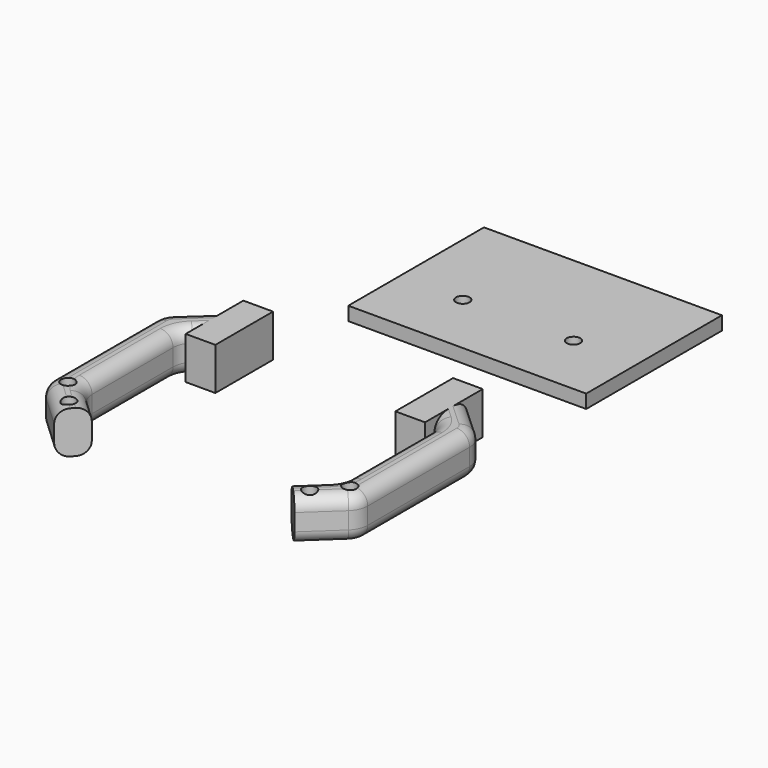
from build123d import *

# Parameters (mm, degrees)
F0_W           = 56.1
F0_H           = 40
F0_R           = 1.6
F1_DEPTH       = 3.2
F2_R           = 1.6
F3_DEPTH       = 10
F4_T1_DEPTH    = 23.8781775711
F4_T3_DEPTH    = 30
F4_T5_DEPTH    = 17.5
F4_T7_DEPTH    = 14.4606096023
F4_T10_ANGLE   = 47.5323400186
F4_T12_ANGLE   = 47.5323400186
F4_T14_ANGLE   = 46.9408390922
F4_T16_ANGLE   = 46.9408390922
F4_T18_ANGLE   = 47.5323400186
F4_T20_ANGLE   = 47.5323400186
F4_T24_DEPTH   = 8.0105146464
F4_T29_DEPTH   = 8.0105146464
F4_T34_DEPTH   = 17.5
F4_T39_DEPTH   = 17.5
F4_T42_ANGLE   = 46.9408390922
F4_T44_ANGLE   = 46.9408390922
F4_2_T1_DEPTH  = 23.8781775711
F4_2_T3_DEPTH  = 30
F4_2_T5_DEPTH  = 14.4606096023
F4_2_T7_DEPTH  = 17.5
F4_2_T12_DEPTH = 8.0105146464
F4_2_T17_DEPTH = 8.0105146464
F4_2_T20_ANGLE = 47.5323400186
F4_2_T22_ANGLE = 47.5323400186
F4_2_T24_ANGLE = 46.9408390922
F4_2_T26_ANGLE = 46.9408390922
F4_2_T28_ANGLE = 47.5323400186
F4_2_T30_ANGLE = 47.5323400186
F4_2_T34_DEPTH = 17.5
F4_2_T39_DEPTH = 17.5
F4_2_T42_ANGLE = 46.9408390922
F4_2_T44_ANGLE = 46.9408390922


# Not quite as in the source:
# - a fillet or chamfer that OpenCascade refuses, or shapes differently, is made with other operations: its cross-section is extruded or revolved along the edge and cut away or added


with BuildPart() as f1:
    # F0 (on Top) → F1 (new body)
    with BuildSketch(Plane.XY):
        with Locations((-11.1600676847, 12.4215162359)):
            Rectangle(F0_W, F0_H)
        with Locations((-24.2100676847, 7.4215162359)):
            Circle(F0_R, mode=Mode.SUBTRACT)
        with Locations((1.8899323153, 7.4215162359)):
            Circle(F0_R, mode=Mode.SUBTRACT)
    extrude(amount=F1_DEPTH)


with BuildPart() as f3:
    # F2 (on Top) → F3 (new body)
    with BuildSketch(Plane.XY):
        with BuildLine():
            Line((-56.4012295696, -43.395672177), (-56.4012295696, -73.395672177))
            ThreePointArc((-56.4012295696, -73.395672177), (-55.9875586538, -75.387049974), (-54.8149953573, -77.0489177403))
            Line((-54.8149953573, -77.0489177403), (-47.5085042306, -83.8764493159))
            Line((-47.5085042306, -83.8764493159), (-42.7292321277, -78.7619055271))
            Line((-42.7292321277, -78.7619055271), (-47.8149953573, -74.0095273427))
            ThreePointArc((-47.8149953573, -74.0095273427), (-48.9875586538, -72.3476595763), (-49.4012295696, -70.3562817793))
            Line((-49.4012295696, -70.3562817793), (-49.4012295696, -46.4781042082))
            ThreePointArc((-49.4012295696, -46.4781042082), (-48.9772184672, -44.4630792435), (-47.7770993263, -42.7898114614))
            Line((-47.7770993263, -42.7898114614), (-47.4005138328, -42.4451252704))
            Line((-47.4005138328, -42.4451252704), (-47.4005138328, -32.9556399168))
            Line((-47.4005138328, -32.9556399168), (-54.7770993263, -39.7073794302))
            ThreePointArc((-54.7770993263, -39.7073794302), (-55.9772184672, -41.3806472123), (-56.4012295696, -43.395672177))
        make_face()
        with Locations((-47.5562252104, -79.4592574239)):
            Circle(F2_R, mode=Mode.SUBTRACT)
        with Locations((-52.413392812, -73.7146958709)):
            Circle(F2_R, mode=Mode.SUBTRACT)
        Polygon((-47.4005138328, -28.2597062046), (-47.4005138328, -32.9556399168), (-47.4005138328, -42.4451252704), (-47.4005138328, -45.2568237537), (-40.4005138328, -45.2568237537), (-40.4005138328, -28.2597062046), align=None)
    extrude(amount=F3_DEPTH)

    # F4: fillet of radius 3 on 18 edges, made by hand

    # F4_s2 → F4_t1 (cut)
    with BuildSketch(Plane.XZ.offset(46.4781042082)):
        with BuildLine():
            ThreePointArc((-49.4012295696, 7), (-50.279909226, 9.1213203436), (-52.4012295696, 10))
            Line((-52.4012295696, 10), (-49.4012295696, 10))
            Line((-49.4012295696, 10), (-49.4012295696, 7))
        make_face()
        with BuildLine():
            ThreePointArc((-49.4012295696, 3), (-50.279909226, 0.8786796564), (-52.4012295696, 0))
            Line((-52.4012295696, 0), (-49.4012295696, 0))
            Line((-49.4012295696, 0), (-49.4012295696, 3))
        make_face()
    extrude(amount=F4_T1_DEPTH, mode=Mode.SUBTRACT)

    # F4_s4 → F4_t3 (cut)
    with BuildSketch(Plane.XZ.offset(43.395672177)):
        with BuildLine():
            ThreePointArc((-56.4012295696, 7), (-55.5225499131, 9.1213203436), (-53.4012295696, 10))
            Line((-53.4012295696, 10), (-56.4012295696, 10))
            Line((-56.4012295696, 10), (-56.4012295696, 7))
        make_face()
        with BuildLine():
            ThreePointArc((-56.4012295696, 3), (-55.5225499131, 0.8786796564), (-53.4012295696, 0))
            Line((-53.4012295696, 0), (-56.4012295696, 0))
            Line((-56.4012295696, 0), (-56.4012295696, 3))
        make_face()
    extrude(amount=F4_T3_DEPTH, mode=Mode.SUBTRACT)

    # F4_s6 → F4_t5 (cut)
    with BuildSketch(Plane(origin=(9.1732003541, -8.571873144, 0), x_dir=(0, 0, 1), z_dir=(0.7306491127, -0.6827531576, 0))):
        with BuildLine():
            ThreePointArc((3, 93.7208345409), (0.8786796564, 92.8421548845), (0, 90.7208345409))
            Line((0, 90.7208345409), (0, 93.7208345409))
            Line((0, 93.7208345409), (3, 93.7208345409))
        make_face()
        with BuildLine():
            ThreePointArc((7, 93.7208345409), (9.1213203436, 92.8421548845), (10, 90.7208345409))
            Line((10, 90.7208345409), (10, 93.7208345409))
            Line((10, 93.7208345409), (7, 93.7208345409))
        make_face()
    extrude(amount=F4_T5_DEPTH, mode=Mode.SUBTRACT)

    # F4_s8 → F4_t7 (cut)
    with BuildSketch(Plane(origin=(21.9595598259, -20.5200534012, 0), x_dir=(0, 0, 1), z_dir=(-0.7306491127, 0.6827531576, 0))):
        with BuildLine():
            ThreePointArc((3, -86.7208345409), (0.8786796564, -87.5995141973), (0, -89.7208345409))
            Line((0, -89.7208345409), (0, -86.7208345409))
            Line((0, -86.7208345409), (3, -86.7208345409))
        make_face()
        with BuildLine():
            ThreePointArc((7, -86.7208345409), (9.1213203436, -87.5995141973), (10, -89.7208345409))
            Line((10, -89.7208345409), (10, -86.7208345409))
            Line((10, -86.7208345409), (7, -86.7208345409))
        make_face()
    extrude(amount=F4_T7_DEPTH, mode=Mode.SUBTRACT)

    # F4_s9 → F4_t10 (revolve, cut)
    with BuildSketch(Plane(origin=(-49.582592704, -45.3826164738, 0), x_dir=(0, 0, 1), z_dir=(0.7376585493, 0.6751739513, 0))):
        with BuildLine():
            ThreePointArc((3, -7.6935826862), (0.8786796564, -6.8149030298), (0, -4.6935826862))
            Line((0, -4.6935826862), (0, -7.6935826862))
            Line((0, -7.6935826862), (3, -7.6935826862))
        make_face()
    revolve(axis=Axis((-51.4012295696, -43.395672177, 0), (0, 0, 1)), revolution_arc=F4_T10_ANGLE, mode=Mode.SUBTRACT)

    # F4_s11 → F4_t12 (revolve, cut)
    with BuildSketch(Plane(origin=(-49.582592704, -45.3826164738, 0), x_dir=(0, 0, 1), z_dir=(0.7376585493, 0.6751739513, 0))):
        with BuildLine():
            ThreePointArc((7, -7.6935826862), (9.1213203436, -6.8149030298), (10, -4.6935826862))
            Line((10, -4.6935826862), (10, -7.6935826862))
            Line((10, -7.6935826862), (7, -7.6935826862))
        make_face()
    revolve(axis=Axis((-51.4012295696, -43.395672177, 10), (0, 0, 1)), revolution_arc=F4_T12_ANGLE, mode=Mode.SUBTRACT)

    # F4_s13 → F4_t14 (revolve, cut)
    with BuildSketch(Plane(origin=(11.3939282512, -10.6470265351, 0), x_dir=(0, 0, 1), z_dir=(0.7306491127, -0.6827531576, 0))):
        with BuildLine():
            ThreePointArc((3, 86.7208345409), (0.8786796564, 87.5995141973), (0, 89.7208345409))
            Line((0, 89.7208345409), (0, 86.7208345409))
            Line((0, 86.7208345409), (3, 86.7208345409))
        make_face()
    revolve(axis=Axis((-44.4012295696, -70.3562817793, 0), (0, 0, -1)), revolution_arc=F4_T14_ANGLE, mode=Mode.SUBTRACT)

    # F4_s15 → F4_t16 (revolve, cut)
    with BuildSketch(Plane(origin=(11.3939282512, -10.6470265351, 0), x_dir=(0, 0, 1), z_dir=(0.7306491127, -0.6827531576, 0))):
        with BuildLine():
            ThreePointArc((7, 86.7208345409), (9.1213203436, 87.5995141973), (10, 89.7208345409))
            Line((10, 89.7208345409), (10, 86.7208345409))
            Line((10, 86.7208345409), (7, 86.7208345409))
        make_face()
    revolve(axis=Axis((-44.4012295696, -70.3562817793, 10), (0, 0, -1)), revolution_arc=F4_T16_ANGLE, mode=Mode.SUBTRACT)

    # F4_s17 → F4_t18 (revolve, cut)
    with BuildSketch(Plane.XZ.offset(46.4781042082)):
        with BuildLine():
            ThreePointArc((-49.4012295696, 3), (-50.279909226, 0.8786796564), (-52.4012295696, 0))
            Line((-52.4012295696, 0), (-49.4012295696, 0))
            Line((-49.4012295696, 0), (-49.4012295696, 3))
        make_face()
    revolve(axis=Axis((-44.4012295696, -46.4781042082, 0), (0, 0, -1)), revolution_arc=F4_T18_ANGLE, mode=Mode.SUBTRACT)

    # F4_s19 → F4_t20 (revolve, cut)
    with BuildSketch(Plane.XZ.offset(46.4781042082)):
        with BuildLine():
            ThreePointArc((-49.4012295696, 7), (-50.279909226, 9.1213203436), (-52.4012295696, 10))
            Line((-52.4012295696, 10), (-49.4012295696, 10))
            Line((-49.4012295696, 10), (-49.4012295696, 7))
        make_face()
    revolve(axis=Axis((-44.4012295696, -46.4781042082, 10), (0, 0, -1)), revolution_arc=F4_T20_ANGLE, mode=Mode.SUBTRACT)


with BuildPart() as f3b:
    # F2 (on Top) → F3, piece 2 (new body)
    with BuildSketch(Plane.XY):
        Polygon((2.0382976284, -45.2568237537), (9.0382976284, -45.2568237537), (9.0382976284, -42.4451252704), (9.0382976284, -32.9556399168), (9.0382976284, -28.2597062046), (2.0382976284, -28.2597062046), align=None)
        with BuildLine():
            Line((9.0382976284, -32.9556399168), (9.0382976284, -42.4451252704))
            Line((9.0382976284, -42.4451252704), (9.4148831219, -42.7898114614))
            ThreePointArc((9.4148831219, -42.7898114614), (10.6150022628, -44.4630792435), (11.0390133652, -46.4781042082))
            Line((11.0390133652, -46.4781042082), (11.0390133652, -70.3562817793))
            ThreePointArc((11.0390133652, -70.3562817793), (10.6253424494, -72.3476595763), (9.4527791529, -74.0095273427))
            Line((9.4527791529, -74.0095273427), (4.3670159233, -78.7619055271))
            Line((4.3670159233, -78.7619055271), (9.1462880262, -83.8764493159))
            Line((9.1462880262, -83.8764493159), (16.4527791529, -77.0489177403))
            ThreePointArc((16.4527791529, -77.0489177403), (17.6253424494, -75.387049974), (18.0390133652, -73.395672177))
            Line((18.0390133652, -73.395672177), (18.0390133652, -43.395672177))
            ThreePointArc((18.0390133652, -43.395672177), (17.6150022628, -41.3806472123), (16.4148831219, -39.7073794302))
            Line((16.4148831219, -39.7073794302), (9.0382976284, -32.9556399168))
        make_face()
        with Locations((9.194009006, -79.4592574239)):
            Circle(F2_R, mode=Mode.SUBTRACT)
        with Locations((14.0511766076, -73.7146958709)):
            Circle(F2_R, mode=Mode.SUBTRACT)
    extrude(amount=F3_DEPTH)

    # F4#2: fillet of radius 3 on 18 edges, made by hand

    # F4_2_s2 → F4_2_t1 (cut)
    with BuildSketch(Plane.XZ.offset(46.4781042082)):
        with BuildLine():
            ThreePointArc((11.0390133652, 7), (11.9176930216, 9.1213203436), (14.0390133652, 10))
            Line((14.0390133652, 10), (11.0390133652, 10))
            Line((11.0390133652, 10), (11.0390133652, 7))
        make_face()
        with BuildLine():
            ThreePointArc((11.0390133652, 3), (11.9176930216, 0.8786796564), (14.0390133652, 0))
            Line((14.0390133652, 0), (11.0390133652, 0))
            Line((11.0390133652, 0), (11.0390133652, 3))
        make_face()
    extrude(amount=F4_2_T1_DEPTH, mode=Mode.SUBTRACT)

    # F4_2_s4 → F4_2_t3 (cut)
    with BuildSketch(Plane.XZ.offset(43.395672177)):
        with BuildLine():
            ThreePointArc((18.0390133652, 7), (17.1603337087, 9.1213203436), (15.0390133652, 10))
            Line((15.0390133652, 10), (18.0390133652, 10))
            Line((18.0390133652, 10), (18.0390133652, 7))
        make_face()
        with BuildLine():
            ThreePointArc((18.0390133652, 3), (17.1603337087, 0.8786796564), (15.0390133652, 0))
            Line((15.0390133652, 0), (18.0390133652, 0))
            Line((18.0390133652, 0), (18.0390133652, 3))
        make_face()
    extrude(amount=F4_2_T3_DEPTH, mode=Mode.SUBTRACT)

    # F4_2_s6 → F4_2_t5 (cut)
    with BuildSketch(Plane(origin=(-31.8735254754, -29.7841327434, 0), x_dir=(0, 0, 1), z_dir=(-0.7306491127, -0.6827531576, 0))):
        with BuildLine():
            ThreePointArc((3, -60.5289102966), (0.8786796564, -61.407589953), (0, -63.5289102966))
            Line((0, -63.5289102966), (0, -60.5289102966))
            Line((0, -60.5289102966), (3, -60.5289102966))
        make_face()
        with BuildLine():
            ThreePointArc((7, -60.5289102966), (9.1213203436, -61.407589953), (10, -63.5289102966))
            Line((10, -63.5289102966), (10, -60.5289102966))
            Line((10, -60.5289102966), (7, -60.5289102966))
        make_face()
    extrude(amount=F4_2_T5_DEPTH, mode=Mode.SUBTRACT)

    # F4_2_s8 → F4_2_t7 (cut)
    with BuildSketch(Plane(origin=(-42.43915705, -39.6571596096, 0), x_dir=(0, 0, 1), z_dir=(0.7306491127, 0.6827531576, 0))):
        with BuildLine():
            ThreePointArc((3, 67.5289102966), (0.8786796564, 66.6502306401), (0, 64.5289102966))
            Line((0, 64.5289102966), (0, 67.5289102966))
            Line((0, 67.5289102966), (3, 67.5289102966))
        make_face()
        with BuildLine():
            ThreePointArc((7, 67.5289102966), (9.1213203436, 66.6502306401), (10, 64.5289102966))
            Line((10, 64.5289102966), (10, 67.5289102966))
            Line((10, 67.5289102966), (7, 67.5289102966))
        make_face()
    extrude(amount=F4_2_T7_DEPTH, mode=Mode.SUBTRACT)


with BuildPart() as f4_tool22:
    # F4_s23 → F4_t24 (new body)
    with BuildSketch(Plane(origin=(-47.3088103634, -43.3014386596, 0), x_dir=(0, 0, 1), z_dir=(0.7376585493, 0.6751739513, 0))):
        with BuildLine():
            ThreePointArc((3, -0.6935826862), (0.8786796564, -1.5722623427), (0, -3.6935826862))
            Line((0, -3.6935826862), (0, -0.6935826862))
            Line((0, -0.6935826862), (3, -0.6935826862))
        make_face()
    extrude(amount=F4_T24_DEPTH)

    split(bisect_by=Plane.YZ.offset(-47.4005138328), keep=Keep.BOTTOM)


with BuildPart() as f3_1:
    add(f3.part)

    # F4_t21: cut F4_tool22
    add(f4_tool22.part, mode=Mode.SUBTRACT)


with BuildPart() as f4_tool27:
    # F4_s28 → F4_t29 (new body)
    with BuildSketch(Plane(origin=(-47.3088103634, -43.3014386596, 0), x_dir=(0, 0, 1), z_dir=(0.7376585493, 0.6751739513, 0))):
        with BuildLine():
            ThreePointArc((7, -0.6935826862), (9.1213203436, -1.5722623427), (10, -3.6935826862))
            Line((10, -3.6935826862), (10, -0.6935826862))
            Line((10, -0.6935826862), (7, -0.6935826862))
        make_face()
    extrude(amount=F4_T29_DEPTH)

    split(bisect_by=Plane.YZ.offset(-47.4005138328), keep=Keep.BOTTOM)


with BuildPart() as f3_2:
    add(f3_1.part)

    # F4_t26: cut F4_tool27
    add(f4_tool27.part, mode=Mode.SUBTRACT)


with BuildPart() as f4_tool32:
    # F4_s33 → F4_t34 (new body)
    with BuildSketch(Plane(origin=(-36.6735680904, -33.5670723253, 0), x_dir=(0, 0, 1), z_dir=(-0.7376585493, -0.6751739513, 0))):
        with BuildLine():
            ThreePointArc((3, 7.6935826862), (0.8786796564, 6.8149030298), (0, 4.6935826862))
            Line((0, 4.6935826862), (0, 7.6935826862))
            Line((0, 7.6935826862), (3, 7.6935826862))
        make_face()
    extrude(amount=F4_T34_DEPTH)

    split(bisect_by=Plane.YZ.offset(-47.4005138328), keep=Keep.BOTTOM)


with BuildPart() as f3_3:
    add(f3_2.part)

    # F4_t31: cut F4_tool32
    add(f4_tool32.part, mode=Mode.SUBTRACT)


with BuildPart() as f4_tool37:
    # F4_s38 → F4_t39 (new body)
    with BuildSketch(Plane(origin=(-36.6735680904, -33.5670723253, 0), x_dir=(0, 0, 1), z_dir=(-0.7376585493, -0.6751739513, 0))):
        with BuildLine():
            ThreePointArc((7, 7.6935826862), (9.1213203436, 6.8149030298), (10, 4.6935826862))
            Line((10, 4.6935826862), (10, 7.6935826862))
            Line((10, 7.6935826862), (7, 7.6935826862))
        make_face()
    extrude(amount=F4_T39_DEPTH)

    split(bisect_by=Plane.YZ.offset(-47.4005138328), keep=Keep.BOTTOM)


with BuildPart() as f3_4:
    add(f3_3.part)

    # F4_t36: cut F4_tool37
    add(f4_tool37.part, mode=Mode.SUBTRACT)

    # F4_s41 → F4_t42 (revolve, cut)
    with BuildSketch(Plane.XZ.offset(73.395672177)):
        with BuildLine():
            ThreePointArc((-56.4012295696, 7), (-55.5225499131, 9.1213203436), (-53.4012295696, 10))
            Line((-53.4012295696, 10), (-56.4012295696, 10))
            Line((-56.4012295696, 10), (-56.4012295696, 7))
        make_face()
    revolve(axis=Axis((-51.4012295696, -73.395672177, 10), (0, 0, 1)), revolution_arc=F4_T42_ANGLE, mode=Mode.SUBTRACT)

    # F4_s43 → F4_t44 (revolve, cut)
    with BuildSketch(Plane.XZ.offset(73.395672177)):
        with BuildLine():
            ThreePointArc((-56.4012295696, 3), (-55.5225499131, 0.8786796564), (-53.4012295696, 0))
            Line((-53.4012295696, 0), (-56.4012295696, 0))
            Line((-56.4012295696, 0), (-56.4012295696, 3))
        make_face()
    revolve(axis=Axis((-51.4012295696, -73.395672177, 0), (0, 0, 1)), revolution_arc=F4_T44_ANGLE, mode=Mode.SUBTRACT)


with BuildPart() as f4_2_tool10:
    # F4_2_s11 → F4_2_t12 (new body)
    with BuildSketch(Plane(origin=(20.525364229, -18.7867290109, 0), x_dir=(0, 0, 1), z_dir=(0.7376585493, -0.6751739513, 0))):
        with BuildLine():
            ThreePointArc((3, 25.2075864107), (0.8786796564, 24.3289067543), (0, 22.2075864107))
            Line((0, 22.2075864107), (0, 25.2075864107))
            Line((0, 25.2075864107), (3, 25.2075864107))
        make_face()
    extrude(amount=F4_2_T12_DEPTH)

    split(bisect_by=Plane.YZ.offset(9.0382976284), keep=Keep.TOP)


with BuildPart() as f3b_1:
    add(f3b.part)

    # F4_2_t9: cut F4_2_tool10
    add(f4_2_tool10.part, mode=Mode.SUBTRACT)


with BuildPart() as f4_2_tool15:
    # F4_2_s16 → F4_2_t17 (new body)
    with BuildSketch(Plane(origin=(20.525364229, -18.7867290109, 0), x_dir=(0, 0, 1), z_dir=(0.7376585493, -0.6751739513, 0))):
        with BuildLine():
            ThreePointArc((7, 25.2075864107), (9.1213203436, 24.3289067543), (10, 22.2075864107))
            Line((10, 22.2075864107), (10, 25.2075864107))
            Line((10, 25.2075864107), (7, 25.2075864107))
        make_face()
    extrude(amount=F4_2_T17_DEPTH)

    split(bisect_by=Plane.YZ.offset(9.0382976284), keep=Keep.TOP)


with BuildPart() as f3b_2:
    add(f3b_1.part)

    # F4_2_t14: cut F4_2_tool15
    add(f4_2_tool15.part, mode=Mode.SUBTRACT)

    # F4_2_s19 → F4_2_t20 (revolve, cut)
    with BuildSketch(Plane(origin=(26.4343888426, -24.195219837, 0), x_dir=(0, 0, 1), z_dir=(-0.7376585493, 0.6751739513, 0))):
        with BuildLine():
            ThreePointArc((3, -25.2075864107), (0.8786796564, -24.3289067543), (0, -22.2075864107))
            Line((0, -22.2075864107), (0, -25.2075864107))
            Line((0, -25.2075864107), (3, -25.2075864107))
        make_face()
    revolve(axis=Axis((6.0390133652, -46.4781042082, 0), (0, 0, -1)), revolution_arc=F4_2_T20_ANGLE, mode=Mode.SUBTRACT)

    # F4_2_s21 → F4_2_t22 (revolve, cut)
    with BuildSketch(Plane(origin=(26.4343888426, -24.195219837, 0), x_dir=(0, 0, 1), z_dir=(-0.7376585493, 0.6751739513, 0))):
        with BuildLine():
            ThreePointArc((7, -25.2075864107), (9.1213203436, -24.3289067543), (10, -22.2075864107))
            Line((10, -22.2075864107), (10, -25.2075864107))
            Line((10, -25.2075864107), (7, -25.2075864107))
        make_face()
    revolve(axis=Axis((6.0390133652, -46.4781042082, 10), (0, 0, -1)), revolution_arc=F4_2_T22_ANGLE, mode=Mode.SUBTRACT)

    # F4_2_s23 → F4_2_t24 (revolve, cut)
    with BuildSketch(Plane.XZ.offset(70.3562817793)):
        with BuildLine():
            ThreePointArc((11.0390133652, 3), (11.9176930216, 0.8786796564), (14.0390133652, 0))
            Line((14.0390133652, 0), (11.0390133652, 0))
            Line((11.0390133652, 0), (11.0390133652, 3))
        make_face()
    revolve(axis=Axis((6.0390133652, -70.3562817793, 0), (0, 0, -1)), revolution_arc=F4_2_T24_ANGLE, mode=Mode.SUBTRACT)

    # F4_2_s25 → F4_2_t26 (revolve, cut)
    with BuildSketch(Plane.XZ.offset(70.3562817793)):
        with BuildLine():
            ThreePointArc((11.0390133652, 7), (11.9176930216, 9.1213203436), (14.0390133652, 10))
            Line((14.0390133652, 10), (11.0390133652, 10))
            Line((11.0390133652, 10), (11.0390133652, 7))
        make_face()
    revolve(axis=Axis((6.0390133652, -70.3562817793, 10), (0, 0, -1)), revolution_arc=F4_2_T26_ANGLE, mode=Mode.SUBTRACT)

    # F4_2_s27 → F4_2_t28 (revolve, cut)
    with BuildSketch(Plane.XZ.offset(43.395672177)):
        with BuildLine():
            ThreePointArc((18.0390133652, 3), (17.1603337087, 0.8786796564), (15.0390133652, 0))
            Line((15.0390133652, 0), (18.0390133652, 0))
            Line((18.0390133652, 0), (18.0390133652, 3))
        make_face()
    revolve(axis=Axis((13.0390133652, -43.395672177, 0), (0, 0, 1)), revolution_arc=F4_2_T28_ANGLE, mode=Mode.SUBTRACT)

    # F4_2_s29 → F4_2_t30 (revolve, cut)
    with BuildSketch(Plane.XZ.offset(43.395672177)):
        with BuildLine():
            ThreePointArc((18.0390133652, 7), (17.1603337087, 9.1213203436), (15.0390133652, 10))
            Line((15.0390133652, 10), (18.0390133652, 10))
            Line((18.0390133652, 10), (18.0390133652, 7))
        make_face()
    revolve(axis=Axis((13.0390133652, -43.395672177, 10), (0, 0, 1)), revolution_arc=F4_2_T30_ANGLE, mode=Mode.SUBTRACT)


with BuildPart() as f4_2_tool32:
    # F4_2_s33 → F4_2_t34 (new body)
    with BuildSketch(Plane(origin=(28.7081711832, -26.2763976513, 0), x_dir=(0, 0, 1), z_dir=(-0.7376585493, 0.6751739513, 0))):
        with BuildLine():
            ThreePointArc((3, -18.2075864107), (0.8786796564, -19.0862660672), (0, -21.2075864107))
            Line((0, -21.2075864107), (0, -18.2075864107))
            Line((0, -18.2075864107), (3, -18.2075864107))
        make_face()
    extrude(amount=F4_2_T34_DEPTH)

    split(bisect_by=Plane.YZ.offset(9.0382976284), keep=Keep.TOP)


with BuildPart() as f3b_3:
    add(f3b_2.part)

    # F4_2_t31: cut F4_2_tool32
    add(f4_2_tool32.part, mode=Mode.SUBTRACT)


with BuildPart() as f4_2_tool37:
    # F4_2_s38 → F4_2_t39 (new body)
    with BuildSketch(Plane(origin=(28.7081711832, -26.2763976513, 0), x_dir=(0, 0, 1), z_dir=(-0.7376585493, 0.6751739513, 0))):
        with BuildLine():
            ThreePointArc((7, -18.2075864107), (9.1213203436, -19.0862660672), (10, -21.2075864107))
            Line((10, -21.2075864107), (10, -18.2075864107))
            Line((10, -18.2075864107), (7, -18.2075864107))
        make_face()
    extrude(amount=F4_2_T39_DEPTH)

    split(bisect_by=Plane.YZ.offset(9.0382976284), keep=Keep.TOP)


with BuildPart() as f3b_4:
    add(f3b_3.part)

    # F4_2_t36: cut F4_2_tool37
    add(f4_2_tool37.part, mode=Mode.SUBTRACT)

    # F4_2_s41 → F4_2_t42 (revolve, cut)
    with BuildSketch(Plane(origin=(-29.6527975783, -27.7089793524, 0), x_dir=(0, 0, 1), z_dir=(-0.7306491127, -0.6827531576, 0))):
        with BuildLine():
            ThreePointArc((7, -67.5289102966), (9.1213203436, -66.6502306401), (10, -64.5289102966))
            Line((10, -64.5289102966), (10, -67.5289102966))
            Line((10, -67.5289102966), (7, -67.5289102966))
        make_face()
    revolve(axis=Axis((13.0390133652, -73.395672177, 10), (0, 0, 1)), revolution_arc=F4_2_T42_ANGLE, mode=Mode.SUBTRACT)

    # F4_2_s43 → F4_2_t44 (revolve, cut)
    with BuildSketch(Plane(origin=(-29.6527975783, -27.7089793524, 0), x_dir=(0, 0, 1), z_dir=(-0.7306491127, -0.6827531576, 0))):
        with BuildLine():
            ThreePointArc((3, -67.5289102966), (0.8786796564, -66.6502306401), (0, -64.5289102966))
            Line((0, -64.5289102966), (0, -67.5289102966))
            Line((0, -67.5289102966), (3, -67.5289102966))
        make_face()
    revolve(axis=Axis((13.0390133652, -73.395672177, 0), (0, 0, 1)), revolution_arc=F4_2_T44_ANGLE, mode=Mode.SUBTRACT)


solid = Compound([f1.part, f3_4.part, f3b_4.part])
